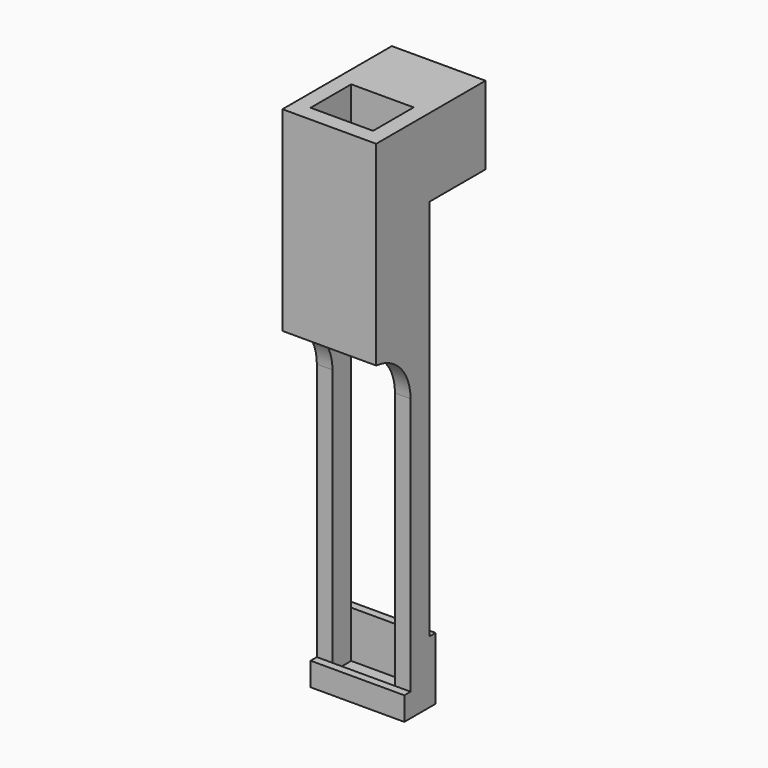
from build123d import *

# Parameters (mm, degrees)
F1_DEPTH     = 16.51
F2_W         = 8.89
F2_H         = 106.68
F3_DEPTH     = 50.8
F4_W         = 5.08
F4_H         = 63.5
F4_W_2       = 25.4
F5_DEPTH     = 5.08
F6_T1_DEPTH  = 5.08
F6_T6_DEPTH  = 43.0474778593
F6_T12_DEPTH = 81.0149557187
F8_DEPTH     = 25.4
F9_W         = 20.32
F9_H         = 15.2493301511
F10_DEPTH    = 2.54
F11_W        = 20.32
F11_H        = 2.54
F12_DEPTH    = 2.54
F13_R        = 0.635
F14_DEPTH    = 2.54
F15_W        = 10.16
F15_H        = 10.16
F15_R        = 0.635
F16_DEPTH    = 1.27


# Not quite as in the source:
# - a fillet or chamfer that OpenCascade refuses, or shapes differently, is made with other operations: its cross-section is extruded or revolved along the edge and cut away or added


with BuildPart() as f1:
    # F0 (on Front) → F1 (new body)
    with BuildSketch(Plane.XZ):
        Polygon((15.24, 6.35), (15.24, 82.55), (10.16, 82.55), (10.16, -82.55), (-10.16, -82.55), (-10.16, 82.55), (-15.24, 82.55), (-15.24, 6.35), (-15.24, -87.63), (15.24, -87.63), align=None)
    extrude(amount=F1_DEPTH)

    # F2 (on face) → F3 (cut)
    with BuildSketch(Plane(origin=(-15.24, 0, 0), x_dir=(0, -1, 0), z_dir=(-1, 0, 0))):
        with Locations((12.065, -34.29)):
            Rectangle(F2_W, F2_H)
    extrude(amount=-F3_DEPTH, mode=Mode.SUBTRACT)

    # F4 (on face) → F5 (join)
    with BuildSketch(Plane.XZ.offset(16.51)):
        with Locations((-12.7, 50.8)):
            Rectangle(F4_W, F4_H)
        with Locations((2.54, 50.8)):
            Rectangle(F4_W_2, F4_H)
    extrude(amount=F5_DEPTH)

    # F6: fillet of radius 15.24 on 1 edges, made by hand

    # F6_s2 → F6_t1 (join)
    with BuildSketch(Plane.YZ.offset(-15.24)):
        with BuildLine():
            ThreePointArc((-21.59, 19.05), (-11.6436636998, 14.1805376301), (-7.62, 3.8630088563))
            Line((-7.62, 3.8630088563), (-7.62, 19.05))
            Line((-7.62, 19.05), (-21.59, 19.05))
        make_face()
    extrude(amount=F6_T1_DEPTH)


with BuildPart() as f6_tool4:
    # F6_s5 → F6_t6 (new body)
    with BuildSketch(Plane.YZ.offset(-15.24)):
        with BuildLine():
            ThreePointArc((-21.59, 19.05), (-11.6436636998, 14.1805376301), (-7.62, 3.8630088563))
            Line((-7.62, 3.8630088563), (-7.62, 19.05))
            Line((-7.62, 19.05), (-21.59, 19.05))
        make_face()
    extrude(amount=F6_T6_DEPTH)

    split(bisect_by=Plane.YZ.offset(15.24), keep=Keep.BOTTOM)

    split(bisect_by=Plane.XZ.offset(16.51), keep=Keep.TOP)


with BuildPart() as f1_1:
    add(f1.part)

    # F6_t3: union F6_tool4
    add(f6_tool4.part)


with BuildPart() as f6_tool10:
    # F6_s11 → F6_t12 (new body)
    with BuildSketch(Plane.YZ.offset(-53.2074778593)):
        with BuildLine():
            ThreePointArc((-21.59, 19.05), (-11.6436636998, 14.1805376301), (-7.62, 3.8630088563))
            Line((-7.62, 3.8630088563), (-7.62, 19.05))
            Line((-7.62, 19.05), (-21.59, 19.05))
        make_face()
    extrude(amount=F6_T12_DEPTH)

    split(bisect_by=Plane.YZ.offset(15.24), keep=Keep.BOTTOM)

    split(bisect_by=Plane.YZ.offset(10.16), keep=Keep.TOP)


with BuildPart() as f1_2:
    add(f1_1.part)

    # F6_t9: union F6_tool10
    add(f6_tool10.part)

    # F7 (on face) → F8 (join)
    with BuildSketch(Plane.XY.offset(82.55)):
        Polygon((10.16, 0), (15.24, 0), (15.24, 22.86), (-15.24, 22.86), (-15.24, 0), (-10.16, 0), align=None)
    extrude(amount=-F8_DEPTH)

    # F9 (on face) → F10 (join)
    with BuildSketch(Plane(origin=(0, 0, 0), x_dir=(-1, 0, 0), z_dir=(0, 1, 0))):
        Polygon((-15.24, -67.3006698489), (-15.24, -87.63), (15.24, -87.63), (15.24, -67.3006698489), (10.16, -67.3006698489), (10.16, -82.55), (-10.16, -82.55), (-10.16, -67.3006698489), align=None)
        with Locations((0, -74.9253349245)):
            Rectangle(F9_W, F9_H)
    extrude(amount=F10_DEPTH)

    # F11 (on face) → F12 (join)
    with BuildSketch(Plane.XZ.offset(7.62)):
        with Locations((0, -81.28)):
            Rectangle(F11_W, F11_H)
        Polygon((-15.24, -80.01), (-15.24, -87.63), (15.24, -87.63), (15.24, -80.01), (10.16, -80.01), (10.16, -82.55), (-10.16, -82.55), (-10.16, -80.01), align=None)
    extrude(amount=F12_DEPTH)

    # F13 (on face) → F14 (cut)
    with BuildSketch(Plane(origin=(0, 22.86, 0), x_dir=(-1, 0, 0), z_dir=(0, 1, 0))):
        with Locations((0, 69.85)):
            Circle(F13_R)
    extrude(amount=-F14_DEPTH, mode=Mode.SUBTRACT)

    # F15 (on face) → F16 (join)
    with BuildSketch(Plane(origin=(0, 22.86, 0), x_dir=(-1, 0, 0), z_dir=(0, 1, 0))):
        with Locations((0, 69.85)):
            Rectangle(F15_W, F15_H)
        with Locations((0, 69.85)):
            Circle(F15_R, mode=Mode.SUBTRACT)
    extrude(amount=F16_DEPTH)


solid = f1_2.part
